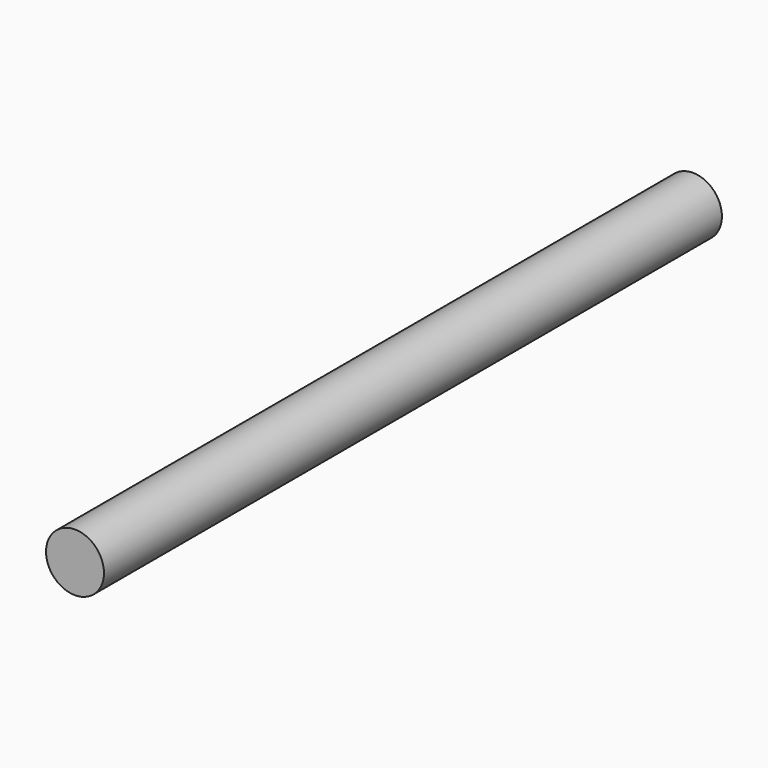
from build123d import *

# Parameters (mm, degrees)
F0_R     = 1.5
F1_DEPTH = 20


with BuildPart() as f1:
    # F0 (on Front) → F1 (new body, symmetric)
    with BuildSketch(Plane.XZ):
        Circle(F0_R)
    extrude(amount=F1_DEPTH, both=True)


solid = f1.part
